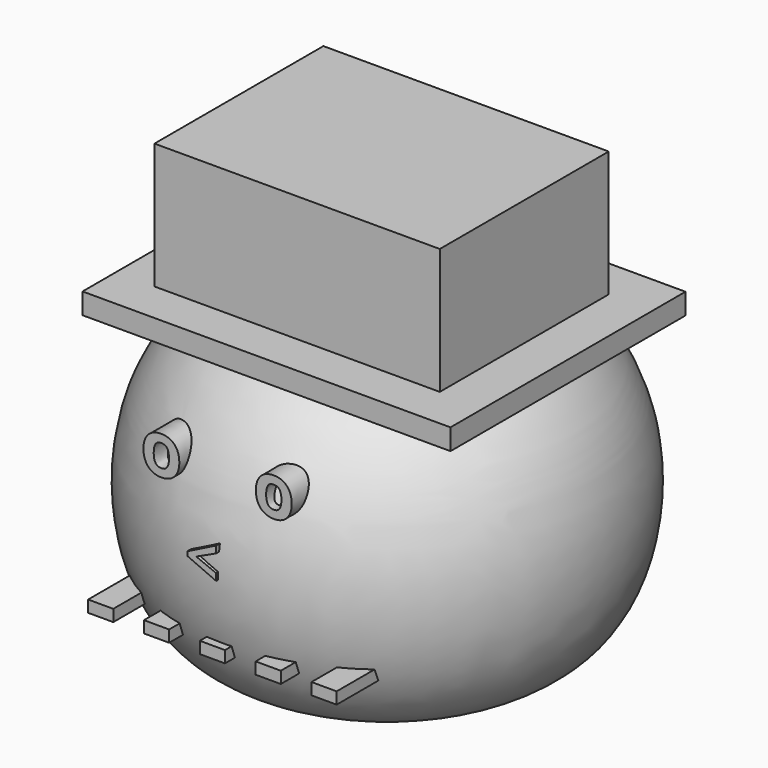
from build123d import *

# Parameters (mm, degrees)
F1_DEPTH      = 10.16
F4_TEXT_SIZE  = 6.5689699517
F5_DEPTH      = 19.812
F6_TEXT_SIZE  = 9.3060390403
F7_DEPTH      = 20.828
F8_W          = 86.710345
F8_H          = 71.5360380709
F8_R          = 25.6053562101
F9_DEPTH      = 84.582
F10_TEXT_SIZE = 5.7478435338
F11_DEPTH     = 21.082
F13_W         = 35.6574002653
F13_H         = 28.467274271
F14_DEPTH     = 2.032
F15_W         = 27.6532266289
F15_H         = 20.4633884132
F16_DEPTH     = 14.224


# Not quite as in the source:
# - Text() gives the source's letters only with a copy of the font that has no kerning and outlines rounded to 1/6400 em; it was checked with that copy


with BuildPart() as f1:
    # F0 (on Front) → F1 (new body)
    with BuildSketch(Plane.XZ):
        with BuildLine():
            add(Edge.make_bspline(
                [(0, 75.6744816899), (3.9020085488, 75.4435725635), (11.9131833667, 74.96949534), (19.9373164543, 63.3312226813), (16.4101441438, 46.3873322148), (5.5220103661, 45.1600247358), (0, 44.5375852287)],
                knots=[0, 0, 0, 0, 0.2308128868, 0.473879635, 0.7331735476, 1, 1, 1, 1], degree=3))
            Line((0, 75.6744816899), (0, 44.5375852287))
        make_face()
    extrude(amount=F1_DEPTH)

    # F1_face (on face) → F3 (revolve)
    with BuildSketch(Plane(origin=(7.9553678844, -10.16, 60.0705039352), x_dir=(1, 0, 0), z_dir=(0, -1, 0))):
        with BuildLine():
            add(Edge.make_bspline(
                [(-7.9553678844, 15.6039777547), (-4.0533593356, 15.3730686283), (3.9578154822, 14.8989914048), (11.9819485698, 3.2607187461), (8.4547762593, -13.6831717205), (-2.4333575183, -14.9104791995), (-7.9553678844, -15.5329187066)],
                knots=[0, 0, 0, 0, 0.2308128868, 0.473879635, 0.7331735476, 1, 1, 1, 1], degree=3))
            Line((-7.9553678844, 15.6039777547), (-7.9553678844, -15.5329187066))
        make_face()
    revolve(axis=Axis((0, 0, 38.0343087018), (0, 0, -1)))

    # F4 (on Front) → F5 (join)
    with BuildSketch(Plane.XZ):
        with Locations((-8.0798277631, 66.0180971026)):
            Text('o    o', F4_TEXT_SIZE, font='Open Sans', font_style=FontStyle.BOLD, text_align=(TextAlign.LEFT, TextAlign.BOTTOM))
    extrude(amount=F5_DEPTH)

    # F8 (on Top) → F9 (cut)
    with BuildSketch(Plane.XY):
        with Locations((0.591205433, -3.6457758397)):
            Rectangle(F8_W, F8_H)
        Circle(F8_R, mode=Mode.SUBTRACT)
    extrude(amount=F9_DEPTH, mode=Mode.SUBTRACT)

    # F13 (on offset) → F14 (join)
    with BuildSketch(Plane.XY.offset(73.914)):
        with Locations((0.0750767067, -0.4930370487)):
            Rectangle(F13_W, F13_H)
    extrude(amount=F14_DEPTH)

    # F15 (on offset) → F16 (join)
    with BuildSketch(Plane.XY.offset(73.914)):
        with Locations((-0.1843543723, -0.4608873278)):
            Rectangle(F15_W, F15_H)
    extrude(amount=F16_DEPTH)


with BuildPart() as f7:
    # F6 (on Front) → F7 (new body)
    with BuildSketch(Plane.XZ):
        with Locations((-12.611920014, 50.841588527)):
            Text('- - - - -', F6_TEXT_SIZE, font='Open Sans', font_style=FontStyle.BOLD, text_align=(TextAlign.LEFT, TextAlign.BOTTOM))
    extrude(amount=F7_DEPTH)


with BuildPart() as f11:
    # F10 (on Front) → F11 (new body)
    with BuildSketch(Plane.XZ):
        with Locations((-2.7589648962, 59.1206923127)):
            Text('<', F10_TEXT_SIZE, font='Open Sans', font_style=FontStyle.BOLD, text_align=(TextAlign.LEFT, TextAlign.BOTTOM))
    extrude(amount=F11_DEPTH)


solid = Compound([f1.part, f7.part, f11.part])
